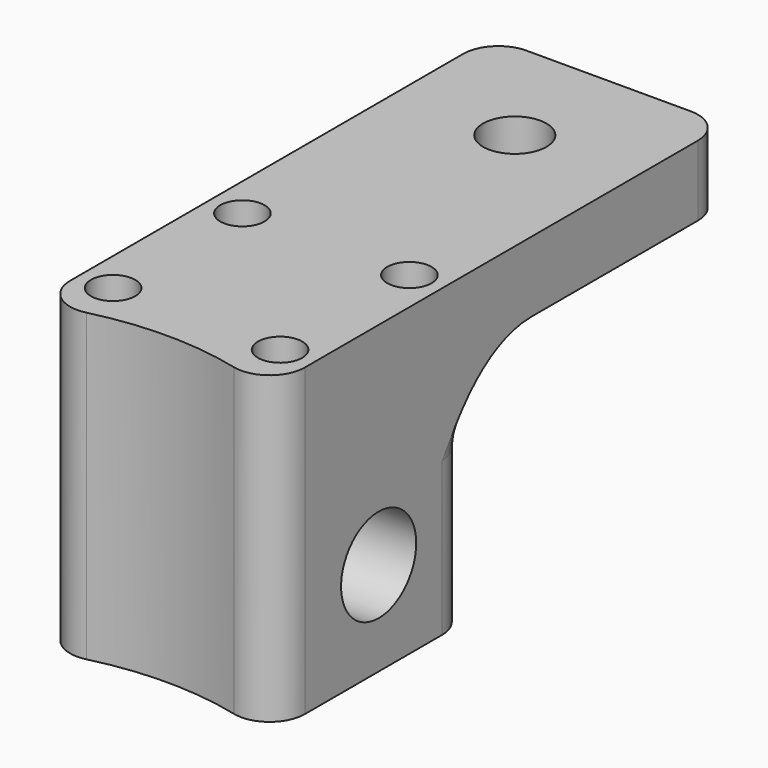
from build123d import *

# Parameters (mm, degrees)
F0_W         = 20
F0_H         = 22.7722101178
F0_R         = 1.8861050589
F0_H_2       = 26.2277898822
F0_R_2       = 2.7
F1_DEPTH     = 6
F2_DEPTH     = 20
F3_R         = 4
F4_DEPTH     = 25
F6_DEPTH     = 20
F7_DEPTH     = 26.001
F8_R         = 3
F9_T2_ANGLE  = 25.7767353783
F9_T6_ANGLE  = 359.64
F9_T11_ANGLE = 359.64


# Not quite as in the source:
# - a fillet or chamfer that OpenCascade refuses, or shapes differently, is made with other operations: its cross-section is extruded or revolved along the edge and cut away or added


with BuildPart() as f1:
    # F0 (on Top) → F1 (new body)
    with BuildSketch(Plane.XY):
        with Locations((0, -13.1138949411)):
            Rectangle(F0_W, F0_H)
        with Locations((-7.1138949411, -19.3861050589)):
            Circle(F0_R, mode=Mode.SUBTRACT)
        with Locations((-7.1138949411, -5.6138949411)):
            Circle(F0_R, mode=Mode.SUBTRACT)
        with Locations((7.1138949411, -19.3861050589)):
            Circle(F0_R, mode=Mode.SUBTRACT)
        with Locations((7.1138949411, -5.6138949411)):
            Circle(F0_R, mode=Mode.SUBTRACT)
        with Locations((0, 11.3861050589)):
            Rectangle(F0_W, F0_H_2)
        with Locations((0, 14.5)):
            Circle(F0_R_2, mode=Mode.SUBTRACT)
    extrude(amount=F1_DEPTH)

    # F0 (on Top) → F2 (join)
    with BuildSketch(Plane.XY):
        with Locations((0, -13.1138949411)):
            Rectangle(F0_W, F0_H)
        with Locations((-7.1138949411, -19.3861050589)):
            Circle(F0_R, mode=Mode.SUBTRACT)
        with Locations((-7.1138949411, -5.6138949411)):
            Circle(F0_R, mode=Mode.SUBTRACT)
        with Locations((7.1138949411, -19.3861050589)):
            Circle(F0_R, mode=Mode.SUBTRACT)
        with Locations((7.1138949411, -5.6138949411)):
            Circle(F0_R, mode=Mode.SUBTRACT)
    extrude(amount=-F2_DEPTH)

    # F3 (on face) → F4 (cut)
    with BuildSketch(Plane.YZ.offset(10)):
        with Locations((-12.5, -12)):
            Circle(F3_R)
    extrude(amount=-F4_DEPTH, mode=Mode.SUBTRACT)

    # F5 (on face) → F6 (cut, through all)
    with BuildSketch(Plane(origin=(0, 0, -20), x_dir=(1, 0, 0), z_dir=(0, 0, -1))):
        with BuildLine():
            Line((-10, 1.7277898822), (10, 1.7277898822))
            ThreePointArc((10, 1.7277898822), (0, 3.5477721311), (-10, 1.7277898822))
        make_face()
    extrude(amount=-F6_DEPTH, mode=Mode.SUBTRACT)

    # F5 (on face) → F7 (cut, through all)
    with BuildSketch(Plane(origin=(0, 0, -20), x_dir=(1, 0, 0), z_dir=(0, 0, -1))):
        with BuildLine():
            ThreePointArc((-10, 24.5), (0, 22.5), (10, 24.5))
            Line((10, 24.5), (-10, 24.5))
        make_face()
    extrude(amount=-F7_DEPTH, mode=Mode.SUBTRACT)

    # F8
    f8_edges = [f1.edges().sort_by_distance(p)[0] for p in [
        (-10, 24.5, 3),
        (10, 24.5, 3),
        (10, -24.5, -7),
        (-10, -24.5, -7),
        (-10, -1.72779, -10),
        (10, -1.72779, -10),
    ]]
    fillet(f8_edges, radius=F8_R)

    # F9: fillet of radius 7 on 1 edges, made by hand

    # F9_s1 → F9_t2 (revolve)
    with BuildSketch(Plane(origin=(5.3999454097, 1.2355988362, 0), x_dir=(0, 0, 1), z_dir=(0.9748064988, 0.2230522133, 0))):
        with BuildLine():
            ThreePointArc((0.0004, -2.8275125891), (-2.0502525317, 2.1232005646), (-7.0009656854, 4.1738530963))
            Line((-7.0009656854, 4.1738530963), (-7.0009656854, 4.8739896648))
            ThreePointArc((-7.0009656854, 4.8739896648), (-3.5004828427, 4.8735896648), (0, 4.8735896648))
            Line((0, 4.8735896648), (0.7001365685, 4.1734530963))
            ThreePointArc((0.7001365685, 4.1734530963), (0.7001365685, 0.6729702536), (0.7005365685, -2.8275125891))
            Line((0.7005365685, -2.8275125891), (0.0004, -2.8275125891))
        make_face()
    revolve(axis=Axis((0, 24.8350144179, 0), (0, 0, -1)), revolution_arc=F9_T2_ANGLE)


with BuildPart() as f9_tool4:
    # F9_s5 → F9_t6 (revolve)
    with BuildSketch(Plane(origin=(5.3999454097, 1.2355988362, 0), x_dir=(0, 0, 1), z_dir=(-0.9748064988, -0.2230522133, 0))):
        with BuildLine():
            ThreePointArc((0.0004, 2.8275125891), (-2.0502525317, -2.1232005646), (-7.0009656854, -4.1738530963))
            Line((-7.0009656854, -4.1738530963), (-7.0009656854, -4.8739896648))
            ThreePointArc((-7.0009656854, -4.8739896648), (-3.5004828427, -4.8735896648), (0, -4.8735896648))
            Line((0, -4.8735896648), (0.7001365685, -4.1734530963))
            ThreePointArc((0.7001365685, -4.1734530963), (0.7001365685, -0.6729702536), (0.7005365685, 2.8275125891))
            Line((0.7005365685, 2.8275125891), (0.0004, 2.8275125891))
        make_face()
    revolve(axis=Axis((7, -5.757129861, 0), (0, 0, -1)), revolution_arc=F9_T6_ANGLE)

    split(bisect_by=Plane.YZ.offset(10), keep=Keep.BOTTOM)


with BuildPart() as f1_1:
    add(f1.part)

    # F9_t3: union F9_tool4
    add(f9_tool4.part)


with BuildPart() as f9_tool9:
    # F9_s10 → F9_t11 (revolve)
    with BuildSketch(Plane(origin=(-5.348096652, 1.2591487889, 0), x_dir=(0, 0, 1), z_dir=(-0.9733857878, 0.22917266, 0))):
        with BuildLine():
            ThreePointArc((0.0004, 2.79284868), (-2.0502525317, -2.1578644738), (-7.0009656854, -4.2085170055))
            Line((-7.0009656854, -4.2085170055), (-7.0009656854, -4.908653574))
            ThreePointArc((-7.0009656854, -4.908653574), (-3.5004828427, -4.908253574), (0, -4.908253574))
            Line((0, -4.908253574), (0.7001365685, -4.2081170055))
            ThreePointArc((0.7001365685, -4.2081170055), (0.7001365685, -0.7076341628), (0.7005365685, 2.79284868))
            Line((0.7005365685, 2.79284868), (0.0004, 2.79284868))
        make_face()
    revolve(axis=Axis((-7, -5.757129861, 0), (0, 0, -1)), revolution_arc=F9_T11_ANGLE)

    split(bisect_by=Plane.YZ.offset(-10), keep=Keep.TOP)


with BuildPart() as f1_2:
    add(f1_1.part)

    # F9_t8: union F9_tool9
    add(f9_tool9.part)


solid = f1_2.part
